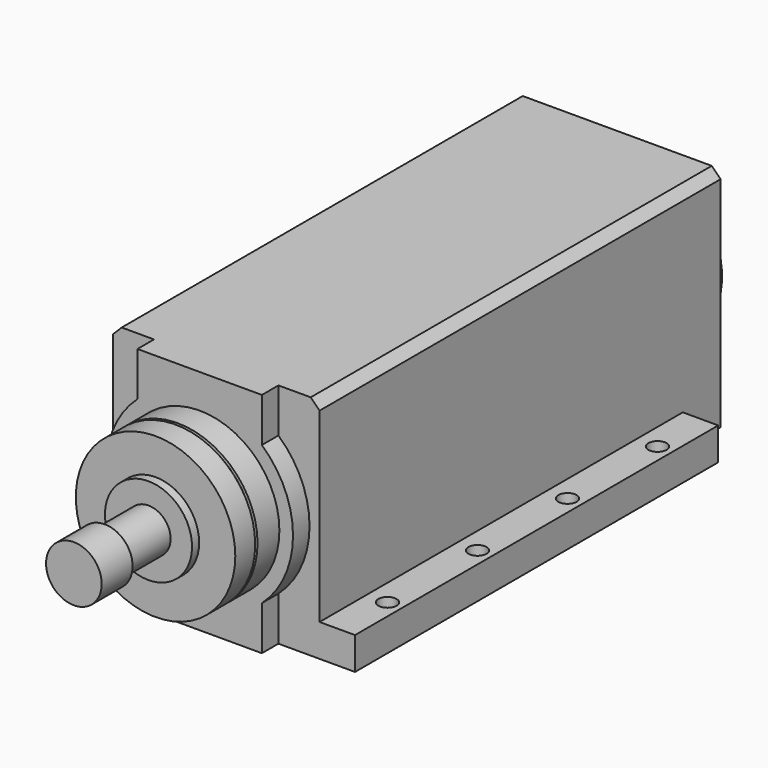
from build123d import *

# Parameters (mm, degrees)
F1_DEPTH  = 153.75
F2_SIZE   = 3
F3_R      = 3.1
F4_DEPTH  = 11.001
F6_DEPTH  = 7
F7_R      = 27
F8_DEPTH  = 18.67
F9_R      = 14.75
F10_DEPTH = 3
F12_W     = 1
F12_H     = 1
F14_R     = 7.5
F15_DEPTH = 18.5
F16_R     = 9.425
F16_R_2   = 7.5
F17_DEPTH = 13.08
F19_DEPTH = 16
F20_R     = 27.5
F21_DEPTH = 10


# Not quite as in the source:
# - the program builds the solid bodies; features that only make, move or delete a surface that nothing else refers to are left out


with BuildPart() as f1:
    # F0 (on Front) → F1 (new body)
    with BuildSketch(Plane.XZ):
        Polygon((0, 11), (0, 0), (94, 0), (94, 11), (82, 11), (82, 77), (12, 77), (12, 11), align=None)
    extrude(amount=F1_DEPTH)

    # F2
    f2_edges = [f1.edges().sort_by_distance(p)[0] for p in [
        (12, -76.875, 77),
        (82, -76.875, 77),
    ]]
    chamfer(f2_edges, length=F2_SIZE)

    # F3 (on face) → F4 (cut, through all)
    with BuildSketch(Plane.XY.offset(11)):
        with Locations((89, -133.75)):
            Circle(F3_R)
        with Locations((89, -95.65)):
            Circle(F3_R)
        with Locations((89, -57.55)):
            Circle(F3_R)
        with Locations((89, -19.45)):
            Circle(F3_R)
        with Locations((5, -19.45)):
            Circle(F3_R)
        with Locations((5, -57.55)):
            Circle(F3_R)
        with Locations((5, -95.65)):
            Circle(F3_R)
        with Locations((5, -133.75)):
            Circle(F3_R)
    extrude(amount=-F4_DEPTH, mode=Mode.SUBTRACT)

    # F5 (on face) → F6 (join)
    with BuildSketch(Plane.XZ.offset(153.75)):
        with BuildLine():
            Line((25.9310321962, 77), (25.9310321962, 62.0646068434))
            ThreePointArc((25.9310321962, 62.0646068434), (15.39, 38.5), (25.9310321962, 14.9353931566))
            Line((25.9310321962, 14.9353931566), (25.9310321962, 0))
            Line((25.9310321962, 0), (68.0689678038, 0))
            Line((68.0689678038, 0), (68.0689678038, 14.9353931566))
            ThreePointArc((68.0689678038, 14.9353931566), (78.61, 38.5), (68.0689678038, 62.0646068434))
            Line((68.0689678038, 62.0646068434), (68.0689678038, 77))
            Line((68.0689678038, 77), (25.9310321962, 77))
        make_face()
    extrude(amount=F6_DEPTH)

    # F7 (on face) → F8 (join)
    with BuildSketch(Plane.XZ.offset(160.75)):
        with Locations((47, 38.5)):
            Circle(F7_R)
    extrude(amount=F8_DEPTH)

    # F9 (on face) → F10 (join)
    with BuildSketch(Plane.XZ.offset(179.42)):
        with Locations((47, 38.5)):
            Circle(F9_R)
    extrude(amount=F10_DEPTH)

    # F12 (on offset) → F13 (revolve, cut)
    with BuildSketch(Plane.YZ.offset(47)):
        with Locations((-170.5, 65)):
            Rectangle(F12_W, F12_H)
    revolve(axis=Axis((47, -160.75, 38.5), (0, 1, 0)), mode=Mode.SUBTRACT)

    # F14 (on face) → F15 (join)
    with BuildSketch(Plane.XZ.offset(182.42)):
        with Locations((47, 38.5)):
            Circle(F14_R)
    extrude(amount=F15_DEPTH)

    # F16 (on face) → F17 (join)
    with BuildSketch(Plane.XZ.offset(200.92)):
        with Locations((47, 38.5)):
            Circle(F16_R)
        with Locations((47, 38.5)):
            Circle(F16_R_2, mode=Mode.SUBTRACT)
        with Locations((47, 38.5)):
            Circle(F16_R_2)
    extrude(amount=F17_DEPTH)

    # F18 (on face) → F19 (join)
    with BuildSketch(Plane(origin=(0, 0, 0), x_dir=(-1, 0, 0), z_dir=(0, 1, 0))):
        Polygon((-79, 77), (-82, 74), (-82, 0), (-12, 0), (-12, 74), (-15, 77), align=None)
    extrude(amount=F19_DEPTH)

    # F20 (on face) → F21 (join)
    with BuildSketch(Plane(origin=(0, 16, 0), x_dir=(-1, 0, 0), z_dir=(0, 1, 0))):
        with Locations((-47, 38.5)):
            Circle(F20_R)
    extrude(amount=F21_DEPTH)


solid = f1.part
